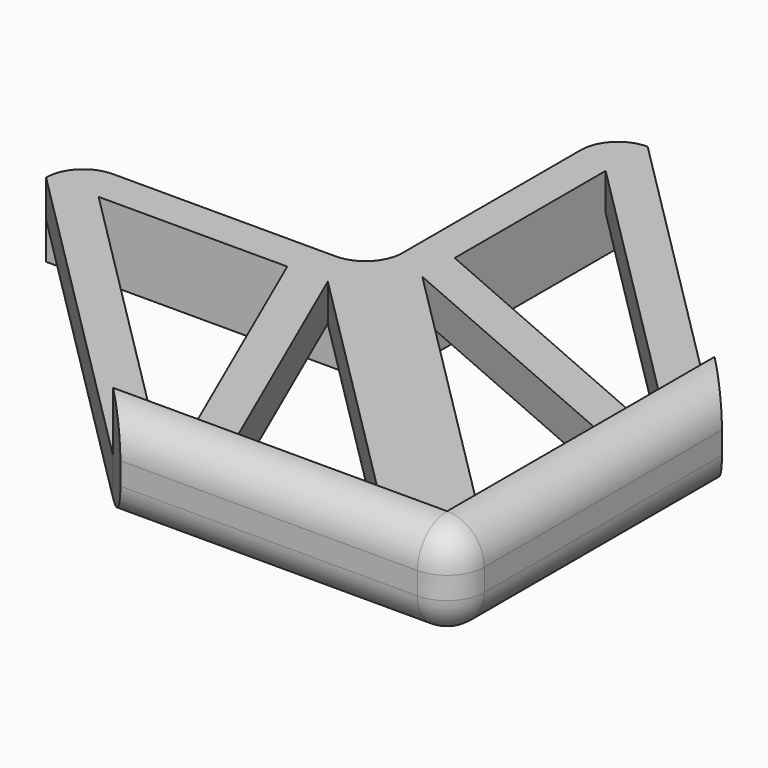
from build123d import *

# Parameters (mm, degrees)
F1_DEPTH  = 5
F3_DEPTH  = 5
F5_DEPTH  = 8
F6_SIZE   = 4.99999
F7_R      = 4.99999
F9_DEPTH  = 5
F11_DEPTH = 5


# Not quite as in the source:
# - a fillet or chamfer is up to 0.001 mm smaller than in the source, because OpenCascade refuses the exact size


with BuildPart() as f1:
    # F0 (on Top) → F1 (new body)
    with BuildSketch(Plane.XY):
        Polygon((0, 45), (-5, 45), (-5, 5), (-45, 5), (-45, 0), (0, -45), (0, -50), (50, -50), (50, 0), (45, 0), align=None)
        Polygon((45, -7.0710678119), (45, -45), (7.0710678119, -45), (-37.9289321881, 0), (0, 0), (0, 37.9289321881), align=None, mode=Mode.SUBTRACT)
    extrude(amount=F1_DEPTH)

    # F2 (on face) → F3 (join)
    with BuildSketch(Plane(origin=(0, 0, 0), x_dir=(1, 0, 0), z_dir=(0, 0, -1))):
        Polygon((0, -45), (0, 0), (-45, 0), (-45, -5), (-5, -5), (-5, -45), align=None)
    extrude(amount=F3_DEPTH)

    # F4 (on face) → F5 (join)
    with BuildSketch(Plane.XY.offset(5)):
        Polygon((50, 0), (45, 0), (45, -45), (0, -45), (0, -50), (50, -50), align=None)
    extrude(amount=F5_DEPTH)

    # F6 (size 5 in the source; OpenCascade refuses exactly that, so slightly less here)
    f6_edges = [f1.edges().sort_by_distance(p)[0] for p in [
        (0, -50, 6.5),
        (50, 0, 6.5),
    ]]
    chamfer(f6_edges, length=F6_SIZE)

    # F7 (radius 5 in the source; OpenCascade refuses exactly that, so slightly less here)
    f7_edges = [f1.edges().sort_by_distance(p)[0] for p in [
        (50, -50, 6.5),
        (-5, 45, 0),
        (-45, 5, 0),
        (-5, 5, 0),
        (50, -27.499995, 13),
        (27.499995, -50, 13),
        (27.499995, -50, 0),
        (50, -27.499995, 0),
    ]]
    fillet(f7_edges, radius=F7_R)

    # F8 (on Top) → F9 (join)
    with BuildSketch(Plane.XY):
        Polygon((0, 0), (-7.0710678119, 0), (37.9289321881, -45), (45, -45), (45, -37.9289321881), (0, 7.0710678119), align=None)
    extrude(amount=F9_DEPTH)

    # F10 (on Top) → F11 (join)
    with BuildSketch(Plane.XY):
        Polygon((45, -7.0710678119), (0, 12.524562237), (0, 7.0710678119), (45, -12.524562237), align=None)
        Polygon((12.524562237, -45), (-7.0710678119, 0), (-12.524562237, 0), (7.0710678119, -45), align=None)
    extrude(amount=F11_DEPTH)


solid = f1.part
